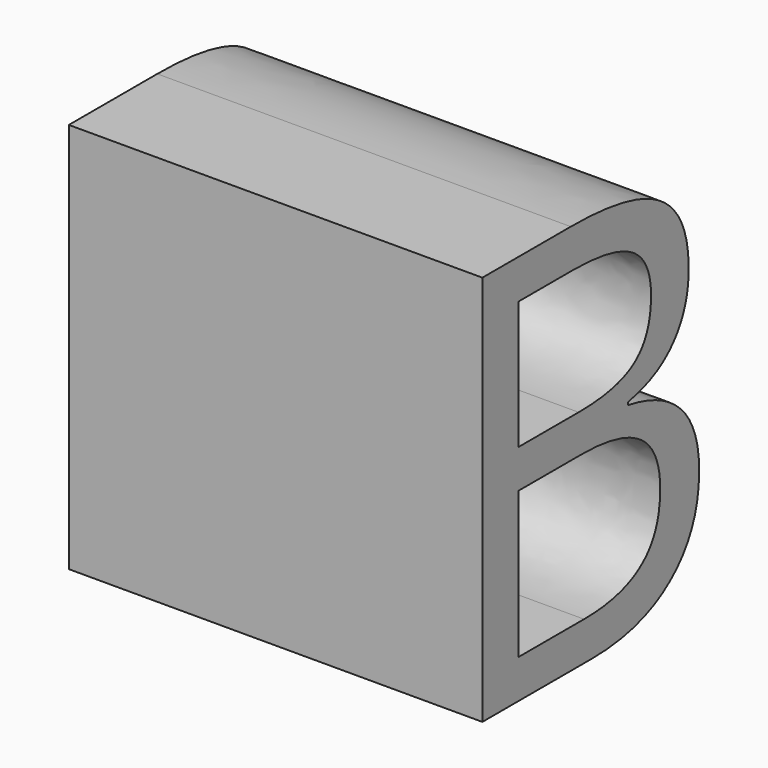
from build123d import *

# Parameters (mm, degrees)
F1_TEXT_SIZE = 104.7059479687
F2_DEPTH     = 79.0370851755


# Not quite as in the source:
# - a feature of the source that left no trace in its solid (it failed there, or was rolled back) is left out
# - Text() gives the source's letters only with a copy of the font that has no kerning and outlines rounded to 1/6400 em; it was checked with that copy


with BuildPart() as f2:
    # F1 (on Right) → F2 (new body)
    with BuildSketch(Plane.YZ):
        with Locations((0, 0)):
            Text('B', F1_TEXT_SIZE, font='Open Sans', text_align=(TextAlign.LEFT, TextAlign.BOTTOM))
    extrude(amount=F2_DEPTH)


solid = f2.part
